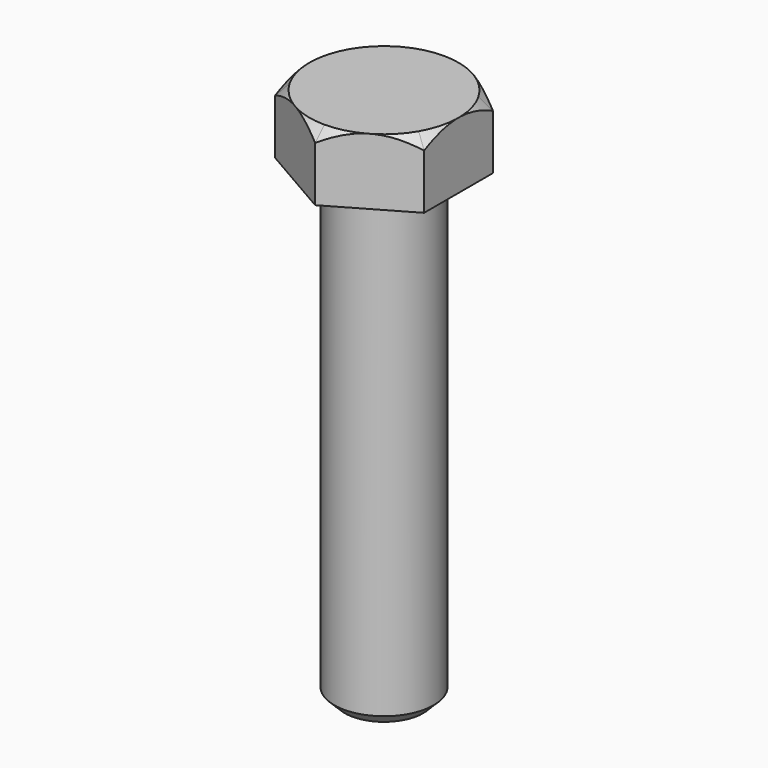
from build123d import *

# Parameters (mm, degrees)
F0_R     = 4.7625
F1_DEPTH = 6.35
F2_SIZE  = 1.1
F3_DEPTH = 6.35
F4_DEPTH = 45
F5_SIZE  = 1


# Not quite as in the source:
# - a length typed as a fraction of an inch, garbled in the dataset ("3 / 203.2 mm" for 3/8 in), is restored


with BuildPart() as f1:
    # F0 (on Top) → F1 (new body)
    with BuildSketch(Plane.XY):
        with BuildLine():
            ThreePointArc((0, -8.248891971), (4.1244459855, -7.14375), (7.14375, -4.1244459855))
            Line((7.14375, -4.1244459855), (0, -8.248891971))
        make_face()
        with BuildLine():
            ThreePointArc((8.248891971, 0), (7.9678177931, 2.1349703431), (7.14375, 4.1244459855))
            Line((7.14375, 4.1244459855), (7.14375, -4.1244459855))
            ThreePointArc((7.14375, -4.1244459855), (7.9678177931, -2.1349703431), (8.248891971, 0))
        make_face()
        with BuildLine():
            Line((0, 8.248891971), (7.14375, 4.1244459855))
            ThreePointArc((7.14375, 4.1244459855), (4.1244459855, 7.14375), (0, 8.248891971))
        make_face()
        with BuildLine():
            Line((-7.14375, 4.1244459855), (0, 8.248891971))
            ThreePointArc((0, 8.248891971), (-4.1244459855, 7.14375), (-7.14375, 4.1244459855))
        make_face()
        Polygon((7.14375, -4.1244459855), (7.14375, 4.1244459855), (0, 8.248891971), (-7.14375, 4.1244459855), (-7.14375, -4.1244459855), (0, -8.248891971), align=None)
        Circle(F0_R, mode=Mode.SUBTRACT)
        Circle(F0_R)
        with BuildLine():
            Line((-7.14375, -4.1244459855), (-7.14375, 4.1244459855))
            ThreePointArc((-7.14375, 4.1244459855), (-8.248891971, 0), (-7.14375, -4.1244459855))
        make_face()
        with BuildLine():
            ThreePointArc((-7.14375, -4.1244459855), (-4.1244459855, -7.14375), (0, -8.248891971))
            Line((0, -8.248891971), (-7.14375, -4.1244459855))
        make_face()
    extrude(amount=F1_DEPTH)

    # F2
    f2_edges = [f1.edges().sort_by_distance(p)[0] for p in [
        (7.14375, 4.124446, 6.35),
    ]]
    chamfer(f2_edges, length=F2_SIZE)

    # F0 (on Top) → F3 (intersect)
    with BuildSketch(Plane.XY):
        Polygon((7.14375, -4.1244459855), (7.14375, 4.1244459855), (0, 8.248891971), (-7.14375, 4.1244459855), (-7.14375, -4.1244459855), (0, -8.248891971), align=None)
        Circle(F0_R, mode=Mode.SUBTRACT)
        Circle(F0_R)
    extrude(amount=F3_DEPTH, mode=Mode.INTERSECT)

    # F0 (on Top) → F4 (join)
    with BuildSketch(Plane.XY):
        Circle(F0_R)
    extrude(amount=-F4_DEPTH)

    # F5
    f5_edges = [f1.edges().sort_by_distance(p)[0] for p in [
        (-4.7625, 0, -45),
    ]]
    chamfer(f5_edges, length=F5_SIZE)


solid = f1.part
